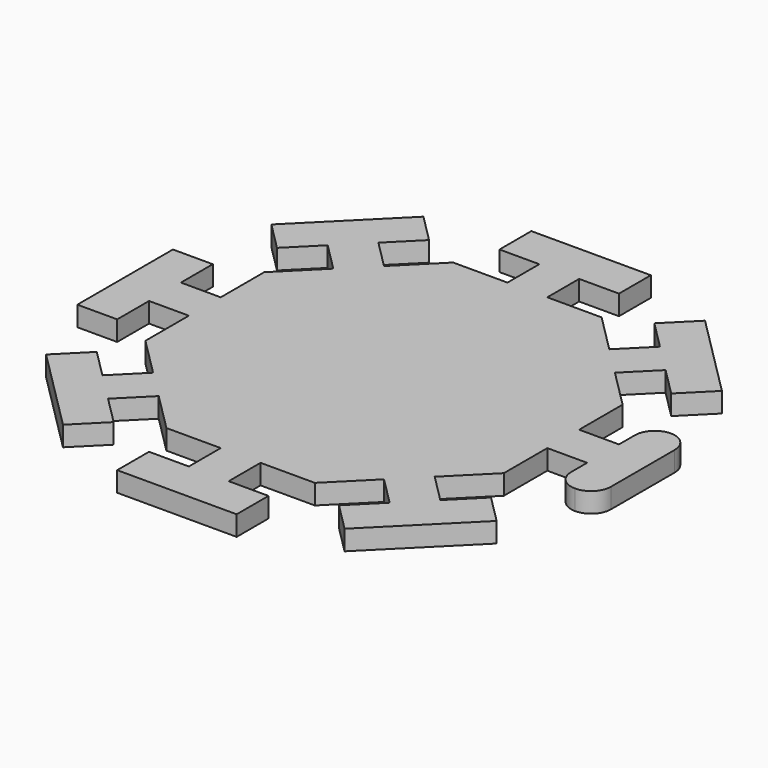
from build123d import *

# Parameters (mm, degrees)
F0_W     = 10
F0_H     = 10
F1_DEPTH = 5
F2_R     = 4.99999


# Not quite as in the source:
# - a fillet or chamfer is up to 0.001 mm smaller than in the source, because OpenCascade refuses the exact size
# - a feature names something its author has since deleted; it is built from what else it names


with BuildPart() as f1:
    # F0 (on Top) → F1 (new body)
    with BuildSketch(Plane.XY):
        Polygon((15, 65), (-15, 65), (-15, 55), (-5, 55), (5, 55), (15, 55), align=None)
        with Locations((0, 50)):
            Rectangle(F0_W, F0_H)
        Polygon((5, 45), (-5, 45), (-18.6396103068, 45), (18.6396103068, -45), (28.2842712475, -35.3553390593), (35.3553390593, -28.2842712475), (45, -18.6396103068), (45, -5), (45, 5), (45, 18.6396103068), (35.3553390593, 28.2842712475), (28.2842712475, 35.3553390593), (18.6396103068, 45), align=None)
        Polygon((18.6396103068, -45), (-18.6396103068, 45), (-28.2842712475, 35.3553390593), (-35.3553390593, 28.2842712475), (-45, 18.6396103068), (-45, 5), (-45, -5), (-45, -18.6396103068), (-35.3553390593, -28.2842712475), (-28.2842712475, -35.3553390593), (-18.6396103068, -45), (-5, -45), (5, -45), align=None)
        Polygon((-35.3553390593, 28.2842712475), (-28.2842712475, 35.3553390593), (-35.3553390593, 42.4264068712), (-42.4264068712, 35.3553390593), align=None)
        Polygon((35.3553390593, 42.4264068712), (28.2842712475, 35.3553390593), (35.3553390593, 28.2842712475), (42.4264068712, 35.3553390593), align=None)
        Polygon((-42.4264068712, 35.3553390593), (-35.3553390593, 42.4264068712), (-28.2842712475, 49.4974746831), (-35.3553390593, 56.5685424949), (-56.5685424949, 35.3553390593), (-49.4974746831, 28.2842712475), align=None)
        with Locations((0, -50)):
            Rectangle(F0_W, F0_H)
        Polygon((35.3553390593, -28.2842712475), (28.2842712475, -35.3553390593), (35.3553390593, -42.4264068712), (42.4264068712, -35.3553390593), align=None)
        Polygon((28.2842712475, 49.4974746831), (35.3553390593, 42.4264068712), (42.4264068712, 35.3553390593), (49.4974746831, 28.2842712475), (56.5685424949, 35.3553390593), (35.3553390593, 56.5685424949), align=None)
        Polygon((15, -55), (5, -55), (-5, -55), (-15, -55), (-15, -65), (15, -65), align=None)
        Polygon((42.4264068712, -35.3553390593), (35.3553390593, -42.4264068712), (28.2842712475, -49.4974746831), (35.3553390593, -56.5685424949), (56.5685424949, -35.3553390593), (49.4974746831, -28.2842712475), align=None)
        with Locations((-50, 0)):
            Rectangle(F0_W, F0_H)
        with Locations((50, 0)):
            Rectangle(F0_W, F0_H)
        Polygon((-55, -5), (-55, 5), (-55, 15), (-65, 15), (-65, -15), (-55, -15), align=None)
        Polygon((-35.3553390593, -42.4264068712), (-28.2842712475, -35.3553390593), (-35.3553390593, -28.2842712475), (-42.4264068712, -35.3553390593), align=None)
        Polygon((55, 15), (55, 5), (55, -5), (55, -15), (65, -15), (65, 15), align=None)
        Polygon((-28.2842712475, -49.4974746831), (-35.3553390593, -42.4264068712), (-42.4264068712, -35.3553390593), (-49.4974746831, -28.2842712475), (-56.5685424949, -35.3553390593), (-35.3553390593, -56.5685424949), align=None)
    extrude(amount=F1_DEPTH)

    # F2 (radius 5 in the source; OpenCascade refuses exactly that, so slightly less here)
    f2_edges = [f1.edges().sort_by_distance(p)[0] for p in [
        (65, 15, 2.5),
        (65, -15, 2.5),
        (55, 15, 2.5),
        (55, -15, 2.5),
    ]]
    fillet(f2_edges, radius=F2_R)


solid = f1.part
